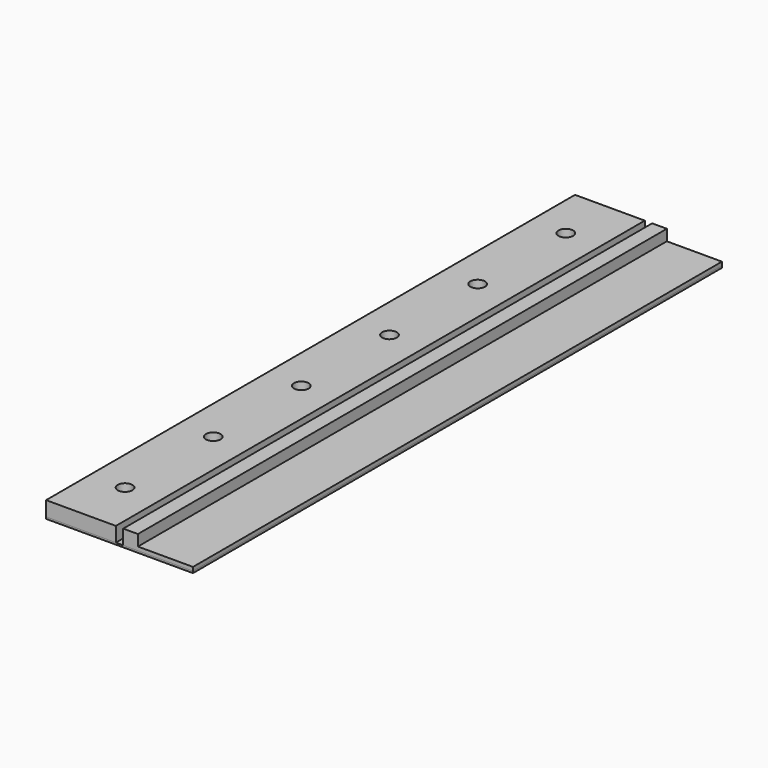
from build123d import *

# Parameters (mm, degrees)
F0_W     = 40
F0_H     = 180
F1_DEPTH = 0.5
F2_W     = 19
F2_H     = 180
F3_DEPTH = 4
F4_W     = 15
F4_H     = 180
F5_DEPTH = 3
F6_R     = 2
F7_DEPTH = 4.501


# Not quite as in the source:
# - a fillet or chamfer that OpenCascade refuses, or shapes differently, is made with other operations: its cross-section is extruded or revolved along the edge and cut away or added


with BuildPart() as f1:
    # F0 (on Top) → F1 (new body)
    with BuildSketch(Plane.XY):
        Rectangle(F0_W, F0_H)
    extrude(amount=F1_DEPTH)


with BuildPart() as f3:
    # F2 (on face) → F3 (new body)
    with BuildSketch(Plane.XY.offset(0.5)):
        with Locations((10.5, 0)):
            Rectangle(F2_W, F2_H)
    extrude(amount=F3_DEPTH)

    # F4 (on face) → F5 (cut)
    with BuildSketch(Plane.XY.offset(4.5)):
        with Locations((12.5, 0)):
            Rectangle(F4_W, F4_H)
    extrude(amount=-F5_DEPTH, mode=Mode.SUBTRACT)


with BuildPart() as f3b:
    # F2 (on face) → F3, piece 2 (new body)
    with BuildSketch(Plane.XY.offset(0.5)):
        with Locations((-10.5, 0)):
            Rectangle(F2_W, F2_H)
    extrude(amount=F3_DEPTH)


with BuildPart() as f7_tool:
    # F6 (on face) → F7 (new body, through all)
    with BuildSketch(Plane.XY.offset(4.5)):
        with Locations((-10.5, 15)):
            Circle(F6_R)
        with Locations((-10.5, 45)):
            Circle(F6_R)
        with Locations((-10.5, 75)):
            Circle(F6_R)
        with Locations((-10.5, -45)):
            Circle(F6_R)
        with Locations((-10.5, -15)):
            Circle(F6_R)
        with Locations((-10.5, -75)):
            Circle(F6_R)
    extrude(amount=-F7_DEPTH)


with BuildPart() as f1_1:
    add(f1.part)

    # F7: cut by f7_tool
    add(f7_tool.part, mode=Mode.SUBTRACT)

    # F8: chamfer of 1 on 6 edges, made by hand

    # F8_s1 → F8_t2 (revolve, cut)
    with BuildSketch(Plane.XZ.offset(75)):
        Polygon((-7.5, 0), (-8.5, 1), (-8.5, 0), align=None)
    revolve(axis=Axis((-10.5, -75, 0), (0, 0, 1)), mode=Mode.SUBTRACT)

    # F8_s3 → F8_t4 (revolve, cut)
    with BuildSketch(Plane.XZ.offset(45)):
        Polygon((-7.5, 0), (-8.5, 1), (-8.5, 0), align=None)
    revolve(axis=Axis((-10.5, -45, 0), (0, 0, 1)), mode=Mode.SUBTRACT)

    # F8_s5 → F8_t6 (revolve, cut)
    with BuildSketch(Plane.XZ.offset(15)):
        Polygon((-7.5, 0), (-8.5, 1), (-8.5, 0), align=None)
    revolve(axis=Axis((-10.5, -15, 0), (0, 0, 1)), mode=Mode.SUBTRACT)

    # F8_s7 → F8_t8 (revolve, cut)
    with BuildSketch(Plane.XZ.offset(-15)):
        Polygon((-7.5, 0), (-8.5, 1), (-8.5, 0), align=None)
    revolve(axis=Axis((-10.5, 15, 0), (0, 0, 1)), mode=Mode.SUBTRACT)

    # F8_s9 → F8_t10 (revolve, cut)
    with BuildSketch(Plane.XZ.offset(-45)):
        Polygon((-7.5, 0), (-8.5, 1), (-8.5, 0), align=None)
    revolve(axis=Axis((-10.5, 45, 0), (0, 0, 1)), mode=Mode.SUBTRACT)

    # F8_s11 → F8_t12 (revolve, cut)
    with BuildSketch(Plane.XZ.offset(-75)):
        Polygon((-7.5, 0), (-8.5, 1), (-8.5, 0), align=None)
    revolve(axis=Axis((-10.5, 75, 0), (0, 0, 1)), mode=Mode.SUBTRACT)


with BuildPart() as f3b_1:
    add(f3b.part)

    # F7: cut by f7_tool
    add(f7_tool.part, mode=Mode.SUBTRACT)


solid = Compound([f3.part, f1_1.part, f3b_1.part])
